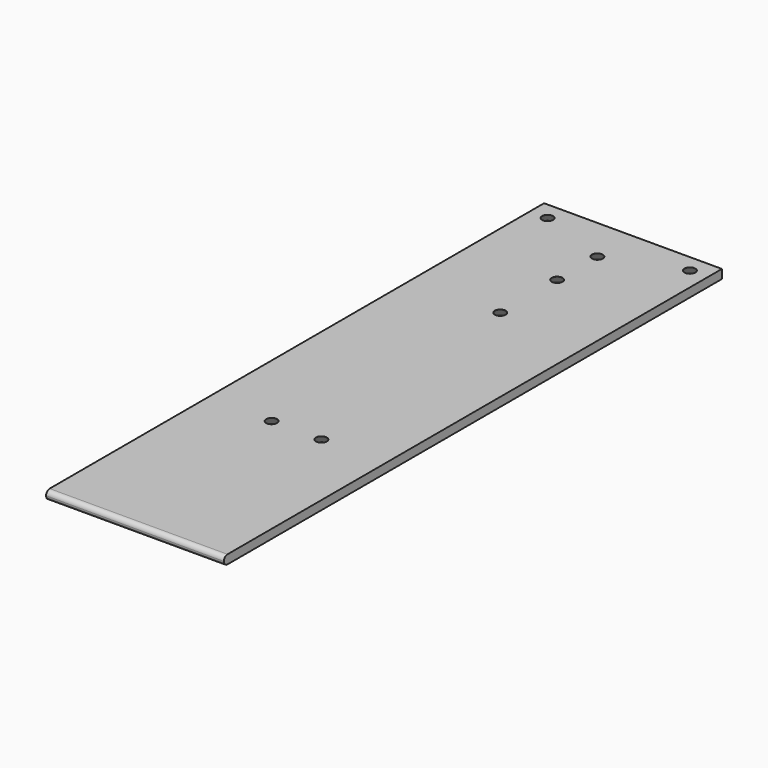
from build123d import *

# Parameters (mm, degrees)
F0_W           = 127
F0_H           = 444.5
F1_DEPTH       = 6.35
F4_D           = 7.7597
F4_DEPTH       = 9.525
F4_CSINK_D     = 17.78
F4_CSINK_ANGLE = 77
F4_TIP         = 2.3312490727
F5_R           = 3.17499


# Not quite as in the source:
# - a fillet or chamfer is up to 0.001 mm smaller than in the source, because OpenCascade refuses the exact size


with BuildPart() as f1:
    # F0 (on Top) → F1 (new body)
    with BuildSketch(Plane.XY):
        with Locations((-9.3688531779, 39.7230851987)):
            Rectangle(F0_W, F0_H)
    extrude(amount=F1_DEPTH)

    # F4
    with Locations(Plane(origin=(0, 0, 0), x_dir=(1, 0, 0), z_dir=(0, 0, -1))):
        with Locations((41.4311468221, -249.2730851987), (-9.3688531779, -230.2230851987), (-60.1688531779, -249.2730851987), (-9.3688531779, -194.2820851987), (-9.3688531779, -143.4820851987), (8.4111468221, 38.3819148013), (-27.1488531779, 38.3819148013)):
            CounterSinkHole(F4_D / 2, F4_CSINK_D / 2, depth=F4_DEPTH, counter_sink_angle=F4_CSINK_ANGLE)
            with Locations((0, 0, -(F4_DEPTH + F4_TIP / 2))):  # 118° drill point
                Cone(0, F4_D / 2, F4_TIP, mode=Mode.SUBTRACT)

    # F5 (radius 3.175 in the source; OpenCascade refuses exactly that, so slightly less here)
    f5_edges = [f1.edges().sort_by_distance(p)[0] for p in [
        (-9.368853, -182.526915, 6.35),
        (-9.368853, -182.526915, 0),
    ]]
    fillet(f5_edges, radius=F5_R)


solid = f1.part
